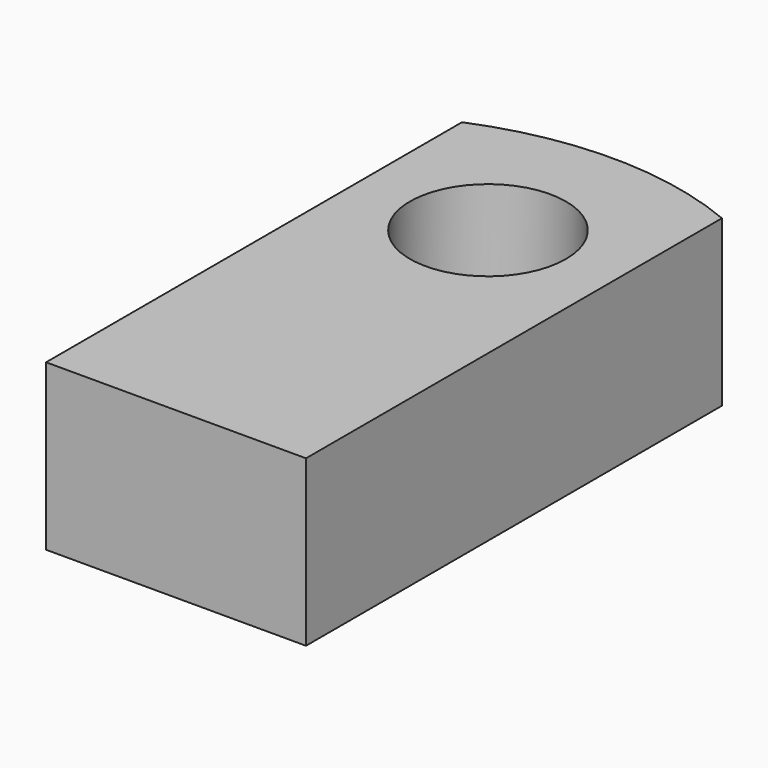
from build123d import *

# Parameters (mm, degrees)
F0_R     = 1.5
F1_DEPTH = 3.175


# Not quite as in the source:
# - a length typed as a fraction of an inch, garbled in the dataset ("3 / 203.2 mm" for 3/8 in), is restored


with BuildPart() as f1:
    # F0 (on Top) → F1 (new body)
    with BuildSketch(Plane.XY):
        with BuildLine():
            Line((-2.5, -5), (2.5, -5))
            Line((2.5, -5), (2.5, 5))
            ThreePointArc((2.5, 5), (0, 5.5), (-2.5, 5))
            Line((-2.5, 5), (-2.5, -5))
        make_face()
        with Locations((0, 2.5)):
            Circle(F0_R, mode=Mode.SUBTRACT)
    extrude(amount=F1_DEPTH)


solid = f1.part
